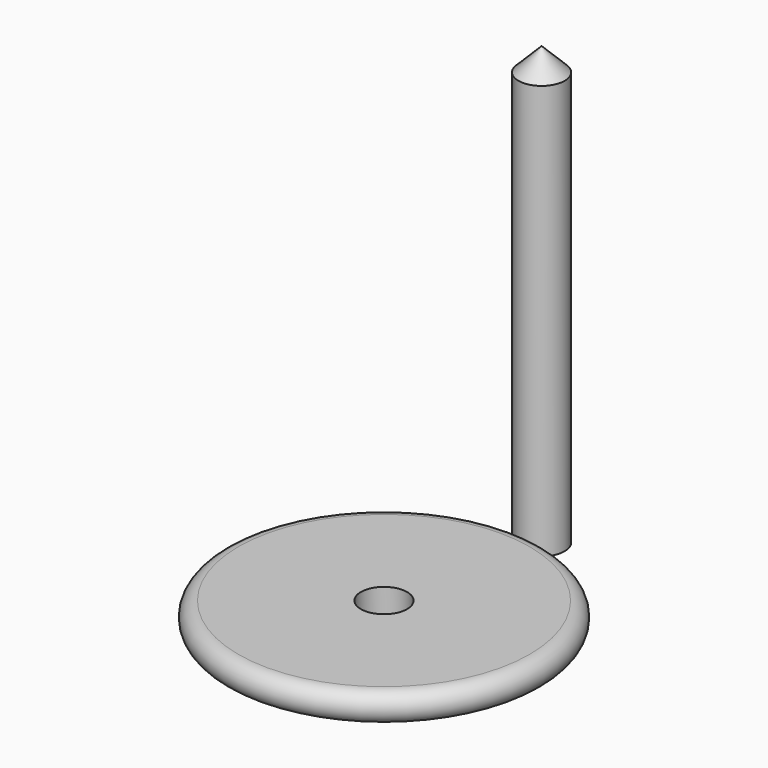
from build123d import *

# Parameters (mm, degrees)
F1_R     = 3.175
F3_DEPTH = 6
F4_R     = 3.175
F5_DEPTH = 60
F6_SIZE  = 3.15


# Not quite as in the source:
# - a feature names something its author has since deleted; it is built from what else it names


with BuildPart() as f2:
    # F0 (on Front) → F2 (revolve)
    with BuildSketch(Plane.XZ):
        with BuildLine():
            Line((0, 4), (0, 0))
            Line((0, 0), (20, 0))
            ThreePointArc((20, 0), (22, 2), (20, 4))
            Line((20, 4), (0, 4))
        make_face()
    revolve(axis=Axis((0, 0, 2), (0, 0, 1)))

    # F1 (on Top) → F3 (cut)
    with BuildSketch(Plane.XY):
        Circle(F1_R)
    extrude(amount=F3_DEPTH, mode=Mode.SUBTRACT)


with BuildPart() as f5:
    # F4 (on Top) → F5 (new body)
    with BuildSketch(Plane.XY):
        with Locations((0, 27.0431211957)):
            Circle(F4_R)
    extrude(amount=F5_DEPTH)

    # F6
    f6_edges = [f5.edges().sort_by_distance(p)[0] for p in [
        (-3.175, 27.043121, 60),
    ]]
    chamfer(f6_edges, length=F6_SIZE)


solid = Compound([f2.part, f5.part])
